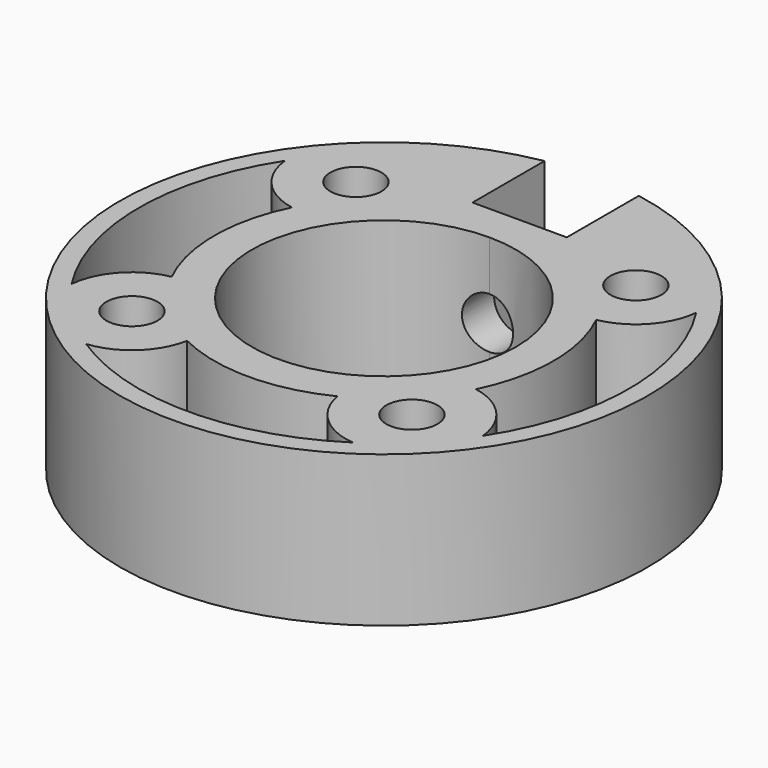
from build123d import *

# Parameters (mm, degrees)
F0_R            = 2.15265
F1_DEPTH        = 12.7
F2_R            = 2.15265
F3_REACH        = 42.6021136501
F5_R            = 3.96875
F6_DEPTH        = 6.35
F8_DEPTH        = 12.7
F8_COPIES_COUNT = 3
F8_COPIES_ANGLE = 180


# Not quite as in the source:
# - a pattern or mirror of a feature is missing from the dataset's text; its kind, count and spacing are read off the source's solid


with BuildPart() as f1:
    # F0 (on Top) → F1 (new body)
    with BuildSketch(Plane.XY):
        with BuildLine():
            Line((3.96875, 14.2875), (0, 14.2875))
            Line((0, 14.2875), (-3.96875, 14.2875))
            Line((-3.96875, 14.2875), (-3.96875, 21.8677764859))
            ThreePointArc((-3.96875, 21.8677764859), (0, -22.225), (3.96875, 21.8677764859))
            Line((3.96875, 21.8677764859), (3.96875, 14.2875))
        make_face()
        with Locations((-11.7865861589, -11.7865861589)):
            Circle(F0_R, mode=Mode.SUBTRACT)
        with Locations((11.7865861589, -11.7865861589)):
            Circle(F0_R, mode=Mode.SUBTRACT)
        with Locations((-11.7865861589, 11.7865861589)):
            Circle(F0_R, mode=Mode.SUBTRACT)
        with BuildLine():
            ThreePointArc((0, 11.1125), (7.8577241059, 7.8577241059), (11.1125, 0))
            ThreePointArc((11.1125, 0), (-7.8577241059, -7.8577241059), (0, 11.1125))
        make_face(mode=Mode.SUBTRACT)
        with Locations((11.7865861589, 11.7865861589)):
            Circle(F0_R, mode=Mode.SUBTRACT)
    extrude(amount=F1_DEPTH)

    f3_end = f1.faces().sort_by_distance((0, -11.1125, 6.35))[0]
    # F2 (on face) → F3 (cut, up to a face of the model that its end follows)
    with BuildSketch(Plane(origin=(0, 14.2875, 0), x_dir=(-1, 0, 0), z_dir=(0, 1, 0))):
        with Locations((0, 6.35)):
            Circle(F2_R)
    f3_long = extrude(amount=-F3_REACH, mode=Mode.PRIVATE)
    add(split(f3_long, bisect_by=f3_end, keep=Keep.ALL, mode=Mode.PRIVATE).solids().sort_by_distance((0, 14.2875, 6.35))[0], mode=Mode.SUBTRACT)

    # F5 (on face) → F6 (cut, through all)
    with BuildSketch(Plane(origin=(0, 0, 0), x_dir=(1, 0, 0), z_dir=(0, 0, -1))):
        with Locations((11.7865861589, -11.7865861589)):
            Circle(F5_R)
        with Locations((-11.7865861589, 11.7865861589)):
            Circle(F5_R)
    extrude(amount=-F6_DEPTH, mode=Mode.SUBTRACT)

    # F7 (on face) → F8 (cut, through all)
    with BuildSketch(Plane(origin=(0, 0, 0), x_dir=(1, 0, 0), z_dir=(0, 0, -1))):
        with BuildLine():
            ThreePointArc((-17.3148424047, -11.229543123), (-15.8788163052, -8.0281867), (-12.8109235396, -6.3255746232))
            ThreePointArc((-12.8109235396, -6.3255746232), (-14.2875, 0), (-12.8109235396, 6.3255746232))
            ThreePointArc((-12.8109235396, 6.3255746232), (-15.8788163052, 8.0281867), (-17.3148424047, 11.229543123))
            ThreePointArc((-17.3148424047, 11.229543123), (-20.6375, 0), (-17.3148424047, -11.229543123))
        make_face()
    f8 = extrude(amount=-F8_DEPTH, mode=Mode.SUBTRACT)

    # F8_copies: F8 ×3 about axis
    f8_copies_axis = Axis((0, 0, 0), (0, 0, 1))
    for i in range(1, F8_COPIES_COUNT):
        add(f8.rotate(f8_copies_axis, i * F8_COPIES_ANGLE / (F8_COPIES_COUNT - 1)), mode=Mode.SUBTRACT)


solid = f1.part
